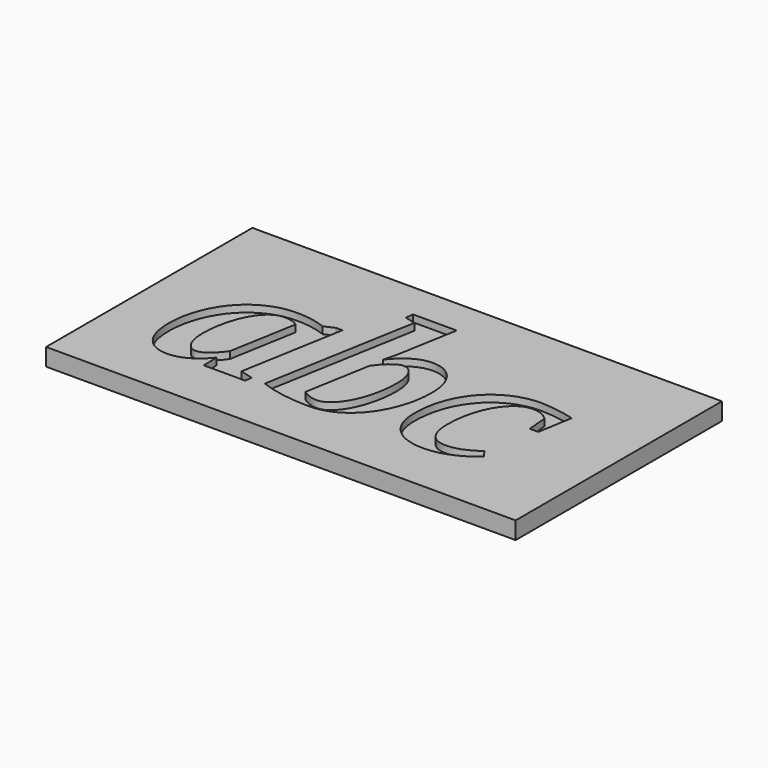
from build123d import *

# Parameters (mm, degrees)
F0_TEXT_SIZE = 89.1603244882
F1_DEPTH     = 2.54
F2_W         = 171.5002134442
F2_H         = 94.1845439374
F3_DEPTH     = 6.35


# Not quite as in the source:
# - Text() gives the source's letters only with a copy of the font that has no kerning and outlines rounded to 1/6400 em; it was checked with that copy


with BuildPart() as f1:
    # F0 (on Top) → F1 (new body)
    with BuildSketch(Plane.XY):
        with Locations((-69.1155232489, -35.7292108238)):
            Text('abc', F0_TEXT_SIZE, font='Tinos', font_style=FontStyle.BOLDITALIC, text_align=(TextAlign.LEFT, TextAlign.BOTTOM))
    extrude(amount=-F1_DEPTH)


with BuildPart() as f3:
    # F2 (on Top) → F3 (new body)
    with BuildSketch(Plane.XY):
        with Locations((-0.4685781896, -7.8487116843)):
            Rectangle(F2_W, F2_H)
    extrude(amount=-F3_DEPTH)

    # F4: cut F1
    add(f1.part, mode=Mode.SUBTRACT)


solid = f3.part
